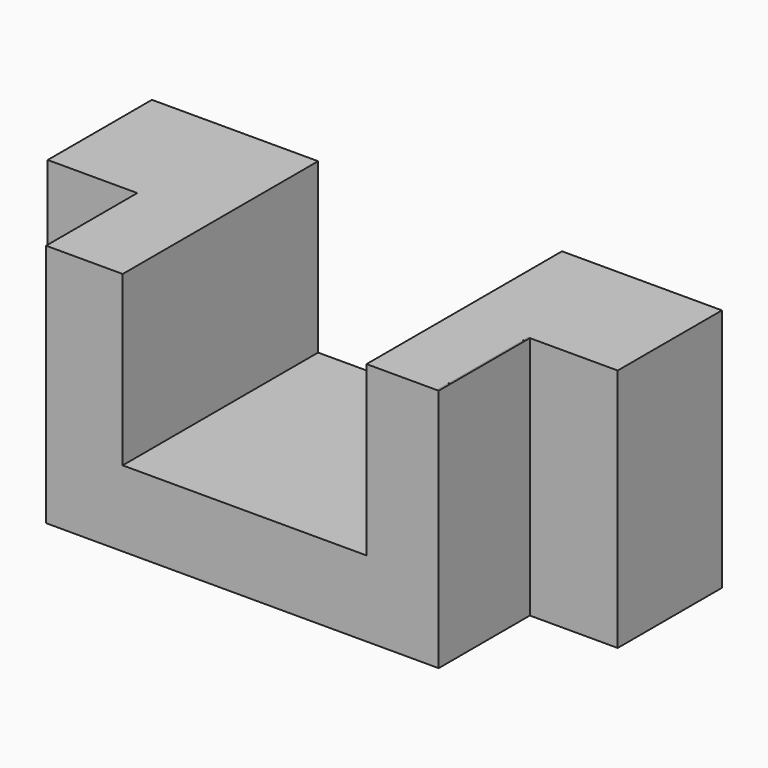
from build123d import *

# Parameters (mm, degrees)
F1_DEPTH = 30
F3_DEPTH = 30


# Not quite as in the source:
# - a feature of the source that left no trace in its solid (it failed there, or was rolled back) is left out


with BuildPart() as f1:
    # F0 (on Top) → F1 (new body)
    with BuildSketch(Plane.XY):
        Polygon((-24.3018865001, 0), (-19.4716978501, 0), (-14.9433972497, 0), (-14.9433972497, 30), (-35.3018865001, 30), (-35.3018865001, 14), (-24.3018865001, 14), align=None)
    extrude(amount=F1_DEPTH)



with BuildPart() as f1b:
    # F0 (on Top) → F1, piece 2 (new body)
    with BuildSketch(Plane.XY):
        Polygon((34.6981134999, 30), (15.0566027503, 30), (15.0566027503, 0), (23.6981134999, 0), (23.6981134999, 14), (34.6981134999, 14), align=None)
    extrude(amount=F1_DEPTH)


with BuildPart() as f1_1:
    add(f1.part)

    add(f1b.part)  # F3 merges F1b
    # F2 (on Front) → F3 (join)
    with BuildSketch(Plane.XZ):
        Polygon((-24.0894670747, 0), (23.9105329253, 0), (23.9105329253, 30), (15.2907075817, 29.9856962232), (15.2907075817, 9.3100926116), (-14.8941018885, 9.3100926116), (-14.8941018885, 30), (-24.0894670747, 30), align=None)
    extrude(amount=-F3_DEPTH)


solid = f1_1.part
